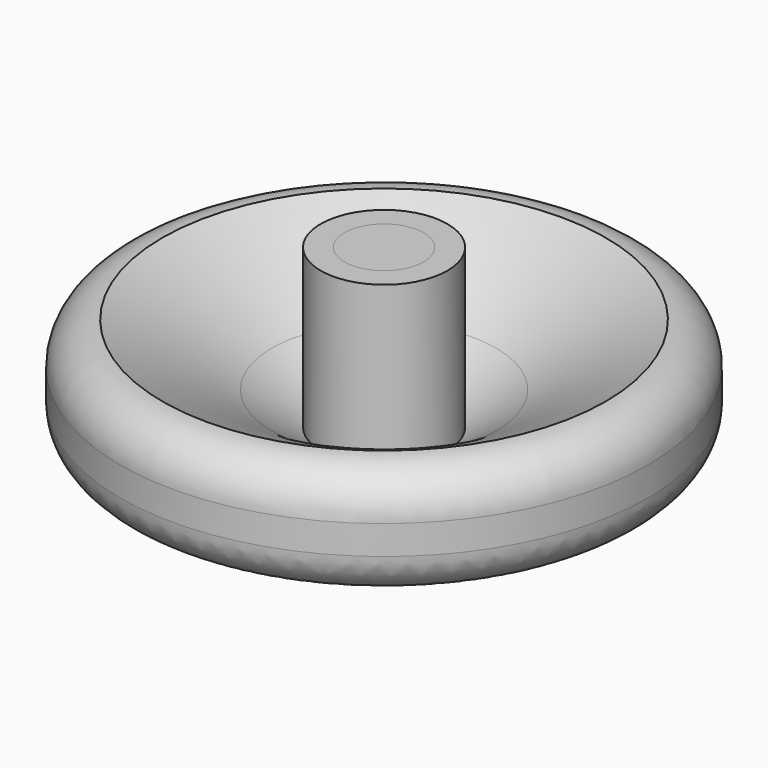
from build123d import *

# Parameters (mm, degrees)
F2_R     = 5.08
F4_R     = 213.36
F5_R     = 4.7625
F6_DEPTH = 9.525
F7_R     = 1.5875
F8_DEPTH = 10.16


# Not quite as in the source:
# - a fillet or chamfer that OpenCascade refuses, or shapes differently, is made with other operations: its cross-section is extruded or revolved along the edge and cut away or added


with BuildPart() as f1:
    # F0 (on Front) → F1 (revolve)
    with BuildSketch(Plane.XZ):
        Polygon((11.9791877568, 4.0159458295), (31.75, 8.134865202), (31.75, 20.834865202), (24.4433090497, 20.834865202), (7.62, 9.4384327507), (7.62, 28.4884327507), (0, 28.4884327507), (0, 0), align=None)
    revolve(axis=Axis((0, 0, 14.2442163754), (0, 0, -1)))

    # F2
    f2_edges = [f1.edges().sort_by_distance(p)[0] for p in [
        (-31.75, 0, 8.134865),
        (-31.75, 0, 20.834865),
        (31.75, 0, 14.484865),
    ]]
    fillet(f2_edges, radius=F2_R)

    # F3: fillet of radius 91.44 on 2 edges, made by hand

    # F3_s1 → F3_t2 (revolve, cut)
    with BuildSketch(Plane.XZ):
        with BuildLine():
            ThreePointArc((26.67, 20.834865202), (19.9318360713, 17.4009600318), (13.5004823618, 13.4219843706))
            Line((13.5004823618, 13.4219843706), (24.4433090497, 20.834865202))
            Line((24.4433090497, 20.834865202), (26.67, 20.834865202))
        make_face()
    revolve(axis=Axis((0, 0, 20.834865202), (0, 0, -1)), mode=Mode.SUBTRACT)

    # F4
    f4_edges = [f1.edges().sort_by_distance(p)[0] for p in [
        (-11.979188, 0, 4.015946),
        (-27.706088, 0, 7.292383),
    ]]
    fillet(f4_edges, radius=F4_R)


with BuildPart() as f6:
    # F5 (on face) → F6 (new body)
    with BuildSketch(Plane.XY.offset(28.4884327507)):
        Circle(F5_R)
    extrude(amount=-F6_DEPTH)


with BuildPart() as f8:
    # F7 (on Top) → F8 (new body)
    with BuildSketch(Plane.XY):
        Circle(F7_R)
    extrude(amount=F8_DEPTH)


solid = Compound([f1.part, f6.part, f8.part])
